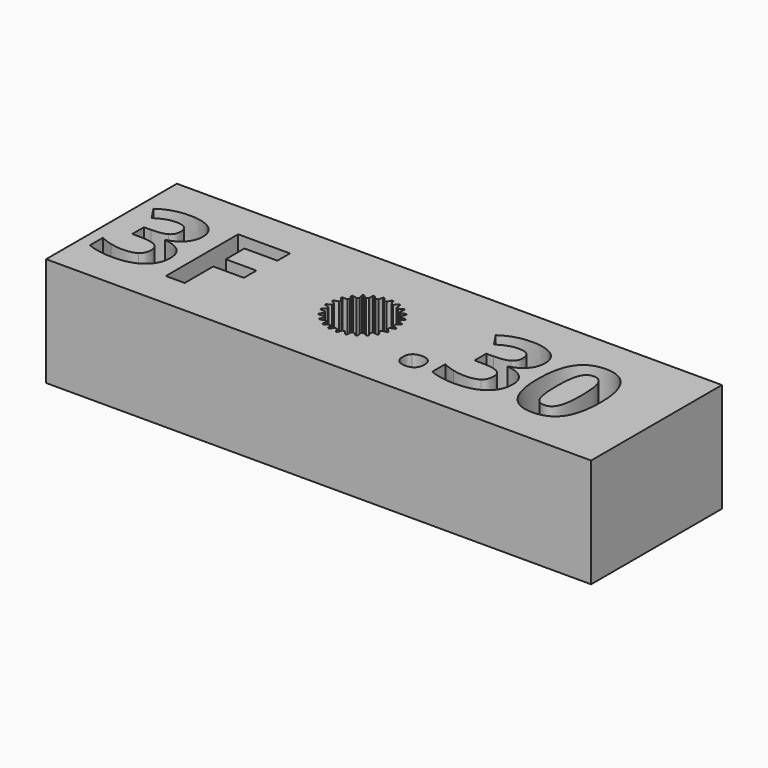
from build123d import *

# Parameters (mm, degrees)
F0_W         = 50
F0_H         = 15
F1_DEPTH     = 10
F0_TEXT_SIZE = 11.6133715069
F2_DEPTH     = 7


# Not quite as in the source:
# - a feature names something its author has since deleted; it is built from what else it names
# - Text() gives the source's letters only with a copy of the font that has no kerning and outlines rounded to 1/6400 em; it was checked with that copy


with BuildPart() as f1:
    # F0 (on Top) → F1 (new body)
    with BuildSketch(Plane.XY):
        with Locations((1.8412548097, 0.1652391267)):
            Rectangle(F0_W, F0_H)
        with BuildLine():
            add(Edge.make_bspline(
                [(-17.3084600185, 3.8715377677), (-16.5626638171, 3.3498433446), (-16.5626638171, 2.420773624)],
                knots=[0, 0, 0, 1, 1, 1], degree=2))
            add(Edge.make_bspline(
                [(-16.5626638171, 2.420773624), (-16.5626638171, 1.6441294045), (-17.0335497399, 1.0997526151)],
                knots=[0, 0, 0, 1, 1, 1], degree=2))
            add(Edge.make_bspline(
                [(-17.0335497399, 1.0997526151), (-17.5044356627, 0.5553758257), (-18.3554780435, 0.3503272351)],
                knots=[0, 0, 0, 1, 1, 1], degree=2))
            Line((-18.3554780435, 0.3503272351), (-18.3554780435, 0.3176646277))
            add(Edge.make_bspline(
                [(-18.3554780435, 0.3176646277), (-17.3501955724, 0.1924579661), (-16.8348522118, -0.2929446711)],
                knots=[0, 0, 0, 1, 1, 1], degree=2))
            add(Edge.make_bspline(
                [(-16.8348522118, -0.2929446711), (-16.3195088512, -0.7783473083), (-16.3195088512, -1.6003562602)],
                knots=[0, 0, 0, 1, 1, 1], degree=2))
            add(Edge.make_bspline(
                [(-16.3195088512, -1.6003562602), (-16.3195088512, -2.7961706076), (-17.1868825356, -3.4630321746)],
                knots=[0, 0, 0, 1, 1, 1], degree=2))
            add(Edge.make_bspline(
                [(-17.1868825356, -3.4630321746), (-18.05425622, -4.1298937416), (-19.6637969273, -4.1298937416)],
                knots=[0, 0, 0, 1, 1, 1], degree=2))
            add(Edge.make_bspline(
                [(-19.6637969273, -4.1298937416), (-21.013851365, -4.1298937416), (-22.0572402113, -3.681690185)],
                knots=[0, 0, 0, 1, 1, 1], degree=2))
            Line((-22.0572402113, -3.681690185), (-22.0572402113, -2.1900977821))
            add(Edge.make_bspline(
                [(-22.0572402113, -2.1900977821), (-21.5763740473, -2.433252748), (-20.9975200613, -2.5865855437)],
                knots=[0, 0, 0, 1, 1, 1], degree=2))
            add(Edge.make_bspline(
                [(-20.9975200613, -2.5865855437), (-20.4186660752, -2.7399183394), (-19.8525142143, -2.7399183394)],
                knots=[0, 0, 0, 1, 1, 1], degree=2))
            add(Edge.make_bspline(
                [(-19.8525142143, -2.7399183394), (-18.9833259406, -2.7399183394), (-18.5695995806, -2.4450475784)],
                knots=[0, 0, 0, 1, 1, 1], degree=2))
            add(Edge.make_bspline(
                [(-18.5695995806, -2.4450475784), (-18.1558732207, -2.1501768175), (-18.1558732207, -1.4969246703)],
                knots=[0, 0, 0, 1, 1, 1], degree=2))
            add(Edge.make_bspline(
                [(-18.1558732207, -1.4969246703), (-18.1558732207, -0.9144415056), (-18.6322029114, -0.670379245)],
                knots=[0, 0, 0, 1, 1, 1], degree=2))
            add(Edge.make_bspline(
                [(-18.6322029114, -0.670379245), (-19.1085326021, -0.4263169845), (-20.1519214484, -0.4263169845)],
                knots=[0, 0, 0, 1, 1, 1], degree=2))
            Line((-20.1519214484, -0.4263169845), (-20.7815839348, -0.4263169845))
            Line((-20.7815839348, -0.4263169845), (-20.7815839348, 0.9182936853))
            Line((-20.7815839348, 0.9182936853), (-20.1410339127, 0.9182936853))
            add(Edge.make_bspline(
                [(-20.1410339127, 0.9182936853), (-19.1774869954, 0.9182936853), (-18.7320053228, 1.1705215977)],
                knots=[0, 0, 0, 1, 1, 1], degree=2))
            add(Edge.make_bspline(
                [(-18.7320053228, 1.1705215977), (-18.2865236501, 1.4227495102), (-18.2865236501, 2.0342661036)],
                knots=[0, 0, 0, 1, 1, 1], degree=2))
            add(Edge.make_bspline(
                [(-18.2865236501, 2.0342661036), (-18.2865236501, 2.9760379492), (-19.4660066938, 2.9760379492)],
                knots=[0, 0, 0, 1, 1, 1], degree=2))
            add(Edge.make_bspline(
                [(-19.4660066938, 2.9760379492), (-19.8742892859, 2.9760379492), (-20.2970885923, 2.8399437519)],
                knots=[0, 0, 0, 1, 1, 1], degree=2))
            add(Edge.make_bspline(
                [(-20.2970885923, 2.8399437519), (-20.7198878987, 2.7038495545), (-21.2352312593, 2.3699651237)],
                knots=[0, 0, 0, 1, 1, 1], degree=2))
            Line((-21.2352312593, 2.3699651237), (-22.0463526755, 3.5766670068))
            add(Edge.make_bspline(
                [(-22.0463526755, 3.5766670068), (-20.9122343643, 4.3932321909), (-19.3408000323, 4.3932321909)],
                knots=[0, 0, 0, 1, 1, 1], degree=2))
            add(Edge.make_bspline(
                [(-19.3408000323, 4.3932321909), (-18.05425622, 4.3932321909), (-17.3084600185, 3.8715377677)],
                knots=[0, 0, 0, 1, 1, 1], degree=2))
        make_face(mode=Mode.SUBTRACT)
        Polygon((-13.0986128473, -0.7384263437), (-13.0986128473, -4.0155746158), (-14.8279164482, -4.0155746158), (-14.8279164482, 4.2752838865), (-10.0755070769, 4.2752838865), (-10.0755070769, 2.834499984), (-13.0986128473, 2.834499984), (-13.0986128473, 0.696913791), (-10.2859994355, 0.696913791), (-10.2859994355, -0.7384263437), align=None, mode=Mode.SUBTRACT)
        with BuildLine():
            ThreePointArc((-0.2085844925, 2.742078137), (-0.1043674356, 2.7480188206), (0, 2.75))
            Line((0, 2.75), (0.2117798247, 3.1428727791))
            ThreePointArc((0.2117798247, 3.1428727791), (0.2764112295, 3.1378490773), (0.3409255665, 3.1314964088))
            Line((0.3409255665, 3.1314964088), (0.4798956754, 2.7078035639))
            ThreePointArc((0.4798956754, 2.7078035639), (0.5823159498, 2.6876398819), (0.6838971897, 2.6636036931))
            Line((0.6838971897, 2.6636036931), (0.9867270488, 2.9914661507))
            ThreePointArc((0.9867270488, 2.9914661507), (1.0480785954, 2.970527101), (1.1089862515, 2.94832995))
            Line((1.1089862515, 2.94832995), (1.1382222331, 2.5033877343))
            ThreePointArc((1.1382222331, 2.5033877343), (1.2324102824, 2.4583866449), (1.3248226038, 2.4098433701))
            Line((1.3248226038, 2.4098433701), (1.6996745836, 2.6520947023))
            ThreePointArc((1.6996745836, 2.6520947023), (1.7538913287, 2.6165559821), (1.8073652517, 2.5799090773))
            Line((1.8073652517, 2.5799090773), (1.7250301017, 2.1416748465))
            ThreePointArc((1.7250301017, 2.1416748465), (1.8050677444, 2.0746639337), (1.8825045413, 2.0046637254))
            Line((1.8825045413, 2.0046637254), (2.3058253134, 2.1460823899))
            ThreePointArc((2.3058253134, 2.1460823899), (2.3495006193, 2.0981770278), (2.3921808461, 2.049383029))
            Line((2.3921808461, 2.049383029), (2.2034479849, 1.6453926516))
            ThreePointArc((2.2034479849, 1.6453926516), (2.2643061615, 1.5605824575), (2.3219017951, 1.4735236862))
            Line((2.3219017951, 1.4735236862), (2.7670925584, 1.5052238283))
            ThreePointArc((2.7670925584, 1.5052238283), (2.7974821452, 1.4479618942), (2.8266869202, 1.3900867079))
            Line((2.8266869202, 1.3900867079), (2.5434151275, 1.045724385))
            ThreePointArc((2.5434151275, 1.045724385), (2.581269895, 0.9484438461), (2.6154054198, 0.8497967345))
            Line((2.6154054198, 0.8497967345), (3.0544932014, 0.7697865177))
            ThreePointArc((3.0544932014, 0.7697865177), (3.0696875795, 0.7067659897), (3.0835818592, 0.6434461265))
            Line((3.0835818592, 0.6434461265), (2.7235701435, 0.3803494094))
            ThreePointArc((2.7235701435, 0.3803494094), (2.7360429477, 0.2767110197), (2.7445735032, 0.1726739287))
            Line((2.7445735032, 0.1726739287), (3.1499688028, -0.0140193109))
            ThreePointArc((3.1499688028, -0.0140193109), (3.1490132537, -0.0788386213), (3.1467240094, -0.1436245414))
            Line((3.1467240094, -0.1436245414), (2.7325932309, -0.3089243183))
            ThreePointArc((2.7325932309, -0.3089243183), (2.7189003595, -0.4124085778), (2.7012899395, -0.5152986151))
            Line((2.7012899395, -0.5152986151), (3.0475202797, -0.7969442547))
            ThreePointArc((3.0475202797, -0.7969442547), (3.0304748438, -0.8594895118), (3.0121459172, -0.9216707511))
            Line((3.0121459172, -0.9216707511), (2.5699174358, -0.9787871951))
            ThreePointArc((2.5699174358, -0.9787871951), (2.5309192623, -1.0756150276), (2.4882743943, -1.1708930518))
            Line((2.4882743943, -1.1708930518), (2.7535848493, -1.5297942599))
            ThreePointArc((2.7535848493, -1.5297942599), (2.7215205542, -1.5861355153), (2.6883036192, -1.6418049979))
            Line((2.6883036192, -1.6418049979), (2.2457642767, -1.5871492726))
            ThreePointArc((2.2457642767, -1.5871492726), (2.1839111998, -1.6712366293), (2.1189114176, -1.7529159718))
            Line((2.1189114176, -1.7529159718), (2.2866315559, -2.1665216656))
            ThreePointArc((2.2866315559, -2.1665216656), (2.2415631192, -2.2131187909), (2.1955453178, -2.2587785986))
            Line((2.1955453178, -2.2587785986), (1.7805014888, -2.0957849242))
            ThreePointArc((1.7805014888, -2.0957849242), (1.6996799648, -2.1618482873), (1.6164094438, -2.2247967345))
            Line((1.6164094438, -2.2247967345), (1.6760007922, -2.6671185472))
            ThreePointArc((1.6760007922, -2.6671185472), (1.6207600295, -2.7010436736), (1.5648328296, -2.7338248326))
            Line((1.5648328296, -2.7338248326), (1.203363244, -2.4727347013))
            ThreePointArc((1.203363244, -2.4727347013), (1.1086515866, -2.5166230666), (1.0123425199, -2.5568853362))
            Line((1.0123425199, -2.5568853362), (0.9600607348, -3.0001305614))
            ThreePointArc((0.9600607348, -3.0001305614), (0.8981186263, -3.0192520486), (0.8357961395, -3.0370947982))
            Line((0.8357961395, -3.0370947982), (0.5506132611, -2.694313463))
            ThreePointArc((0.5506132611, -2.694313463), (0.4479625518, -2.7132691632), (0.3446663923, -2.7283154286))
            Line((0.3446663923, -2.7283154286), (0.1837965306, -3.1446333388))
            ThreePointArc((0.1837965306, -3.1446333388), (0.1190451269, -3.1477497133), (0.0542433042, -3.1495329279))
            Line((0.0542433042, -3.1495329279), (-0.1367337781, -2.7465986008))
            ThreePointArc((-0.1367337781, -2.7465986008), (-0.2408736175, -2.7394305796), (-0.3446663923, -2.7283154286))
            Line((-0.3446663923, -2.7283154286), (-0.6040162856, -3.0915472383))
            ThreePointArc((-0.6040162856, -3.0915472383), (-0.6675084157, -3.078462687), (-0.7307178374, -3.0640743206))
            Line((-0.7307178374, -3.0640743206), (-0.8154893312, -2.6263048473))
            ThreePointArc((-0.8154893312, -2.6263048473), (-0.9145748116, -2.5934634977), (-1.0123425199, -2.5568853362))
            Line((-1.0123425199, -2.5568853362), (-1.3538765371, -2.844207855))
            ThreePointArc((-1.3538765371, -2.844207855), (-1.4121199496, -2.8157445282), (-1.4697652899, -2.7860886548))
            Line((-1.4697652899, -2.7860886548), (-1.4430046904, -2.3409907013))
            ThreePointArc((-1.4430046904, -2.3409907013), (-1.5308099067, -2.2845395662), (-1.6164094438, -2.2247967345))
            Line((-1.6164094438, -2.2247967345), (-2.0186677466, -2.4181564318))
            ThreePointArc((-2.0186677466, -2.4181564318), (-2.0680027937, -2.3761027851), (-2.1164619838, -2.3330427924))
            Line((-2.1164619838, -2.3330427924), (-1.9798507579, -1.9085835))
            ThreePointArc((-1.9798507579, -1.9085835), (-2.0508585855, -1.8320696117), (-2.1189114176, -1.7529159718))
            Line((-2.1189114176, -1.7529159718), (-2.5566186375, -1.8401633467))
            ThreePointArc((-2.5566186375, -1.8401633467), (-2.5939454167, -1.7871617653), (-2.6301735875, -1.733403271))
            Line((-2.6301735875, -1.733403271), (-2.3922955209, -1.3562529781))
            ThreePointArc((-2.3922955209, -1.3562529781), (-2.4420442768, -1.2644839857), (-2.4882743943, -1.1708930518))
            Line((-2.4882743943, -1.1708930518), (-2.9339277767, -1.1465460309))
            ThreePointArc((-2.9339277767, -1.1465460309), (-2.9569009092, -1.0859267991), (-2.9786217115, -1.024847647))
            Line((-2.9786217115, -1.024847647), (-2.6544235581, -0.7187040937))
            ThreePointArc((-2.6544235581, -0.7187040937), (-2.679787345, -0.6174461804), (-2.7012899395, -0.5152986151))
            Line((-2.7012899395, -0.5152986151), (-3.1268874436, -0.3808870112))
            ThreePointArc((-3.1268874436, -0.3808870112), (-3.1340634429, -0.3164590584), (-3.1399120789, -0.2518970763))
            Line((-3.1399120789, -0.2518970763), (-2.7497644008, -0.0359963878))
            ThreePointArc((-2.7497644008, -0.0359963878), (-2.7491495187, 0.0683880392), (-2.7445735032, 0.1726739287))
            Line((-2.7445735032, 0.1726739287), (-3.1233732724, 0.4087045402))
            ThreePointArc((-3.1233732724, 0.4087045402), (-3.1143012443, 0.4728929689), (-3.1039102225, 0.5368811142))
            Line((-3.1039102225, 0.5368811142), (-2.6723274333, 0.6489731035))
            ThreePointArc((-2.6723274333, 0.6489731035), (-2.6457725175, 0.7499251868), (-2.6154054198, 0.8497967345))
            Line((-2.6154054198, 0.8497967345), (-2.9236060716, 1.1726156822))
            ThreePointArc((-2.9236060716, 1.1726156822), (-2.8988560448, 1.2325313917), (-2.8728782714, 1.2919250897))
            Line((-2.8728782714, 1.2919250897), (-2.4269783051, 1.2931652279))
            ThreePointArc((-2.4269783051, 1.2931652279), (-2.3761518985, 1.3843417768), (-2.3219017951, 1.4735236862))
            Line((-2.3219017951, 1.4735236862), (-2.540137949, 1.8628470683))
            ThreePointArc((-2.540137949, 1.8628470683), (-2.5012650588, 1.9147253343), (-2.4613328129, 1.9657926605))
            Line((-2.4613328129, 1.9657926605), (-2.0291332041, 1.8561030252))
            ThreePointArc((-2.0291332041, 1.8561030252), (-1.9572289169, 1.9317750818), (-1.8825045413, 2.0046637254))
            Line((-1.8825045413, 2.0046637254), (-1.9970636172, 2.436028922))
            ThreePointArc((-1.9970636172, 2.436028922), (-1.9465103901, 2.4766100422), (-1.8951327616, 2.5161422488))
            Line((-1.8951327616, 2.5161422488), (-1.5037902013, 2.3024150431))
            ThreePointArc((-1.5037902013, 2.3024150431), (-1.4153260443, 2.3578278538), (-1.3248226038, 2.4098433701))
            Line((-1.3248226038, 2.4098433701), (-1.3285064335, 2.8561461195))
            ThreePointArc((-1.3285064335, 2.8561461195), (-1.2694493149, 2.8828802328), (-1.209854549, 2.9083933658))
            Line((-1.209854549, 2.9083933658), (-0.8839585296, 2.6040578561))
            ThreePointArc((-0.8839585296, 2.6040578561), (-0.7844930311, 2.6357296303), (-0.6838971897, 2.6636036931))
            Line((-0.6838971897, 2.6636036931), (-0.5764743048, 3.0968011521))
            ThreePointArc((-0.5764743048, 3.0968011521), (-0.5126240705, 3.108008456), (-0.4485567256, 3.1178994313))
            Line((-0.4485567256, 3.1178994313), (-0.2085844925, 2.742078137))
        make_face(mode=Mode.SUBTRACT)
        with BuildLine():
            add(Edge.make_bspline(
                [(6.516190169, -3.9157722044), (6.2557966047, -3.663544292), (6.2557966047, -3.2044531996)],
                knots=[0, 0, 0, 1, 1, 1], degree=2))
            add(Edge.make_bspline(
                [(6.2557966047, -3.2044531996), (6.2557966047, -2.7290308036), (6.5107464011, -2.484968543)],
                knots=[0, 0, 0, 1, 1, 1], degree=2))
            add(Edge.make_bspline(
                [(6.5107464011, -2.484968543), (6.7656961974, -2.2409062824), (7.2538207186, -2.2409062824)],
                knots=[0, 0, 0, 1, 1, 1], degree=2))
            add(Edge.make_bspline(
                [(7.2538207186, -2.2409062824), (7.7237993467, -2.2409062824), (7.9814710271, -2.4904123109)],
                knots=[0, 0, 0, 1, 1, 1], degree=2))
            add(Edge.make_bspline(
                [(7.9814710271, -2.4904123109), (8.2391427074, -2.7399183394), (8.2391427074, -3.2044531996)],
                knots=[0, 0, 0, 1, 1, 1], degree=2))
            add(Edge.make_bspline(
                [(8.2391427074, -3.2044531996), (8.2391427074, -3.6526567562), (7.9787491431, -3.9103284365)],
                knots=[0, 0, 0, 1, 1, 1], degree=2))
            add(Edge.make_bspline(
                [(7.9787491431, -3.9103284365), (7.7183555789, -4.1680001168), (7.2538207186, -4.1680001168)],
                knots=[0, 0, 0, 1, 1, 1], degree=2))
            add(Edge.make_bspline(
                [(7.2538207186, -4.1680001168), (6.7765837332, -4.1680001168), (6.516190169, -3.9157722044)],
                knots=[0, 0, 0, 1, 1, 1], degree=2))
        make_face(mode=Mode.SUBTRACT)
        with BuildLine():
            add(Edge.make_bspline(
                [(14.0948223719, 3.8715377677), (14.8406185733, 3.3498433446), (14.8406185733, 2.420773624)],
                knots=[0, 0, 0, 1, 1, 1], degree=2))
            add(Edge.make_bspline(
                [(14.8406185733, 2.420773624), (14.8406185733, 1.6441294045), (14.3697326505, 1.0997526151)],
                knots=[0, 0, 0, 1, 1, 1], degree=2))
            add(Edge.make_bspline(
                [(14.3697326505, 1.0997526151), (13.8988467277, 0.5553758257), (13.0478043469, 0.3503272351)],
                knots=[0, 0, 0, 1, 1, 1], degree=2))
            Line((13.0478043469, 0.3503272351), (13.0478043469, 0.3176646277))
            add(Edge.make_bspline(
                [(13.0478043469, 0.3176646277), (14.053086818, 0.1924579661), (14.5684301786, -0.2929446711)],
                knots=[0, 0, 0, 1, 1, 1], degree=2))
            add(Edge.make_bspline(
                [(14.5684301786, -0.2929446711), (15.0837735393, -0.7783473083), (15.0837735393, -1.6003562602)],
                knots=[0, 0, 0, 1, 1, 1], degree=2))
            add(Edge.make_bspline(
                [(15.0837735393, -1.6003562602), (15.0837735393, -2.7961706076), (14.2163998548, -3.4630321746)],
                knots=[0, 0, 0, 1, 1, 1], degree=2))
            add(Edge.make_bspline(
                [(14.2163998548, -3.4630321746), (13.3490261704, -4.1298937416), (11.7394854631, -4.1298937416)],
                knots=[0, 0, 0, 1, 1, 1], degree=2))
            add(Edge.make_bspline(
                [(11.7394854631, -4.1298937416), (10.3894310254, -4.1298937416), (9.3460421791, -3.681690185)],
                knots=[0, 0, 0, 1, 1, 1], degree=2))
            Line((9.3460421791, -3.681690185), (9.3460421791, -2.1900977821))
            add(Edge.make_bspline(
                [(9.3460421791, -2.1900977821), (9.8269083431, -2.433252748), (10.4057623291, -2.5865855437)],
                knots=[0, 0, 0, 1, 1, 1], degree=2))
            add(Edge.make_bspline(
                [(10.4057623291, -2.5865855437), (10.9846163152, -2.7399183394), (11.5507681761, -2.7399183394)],
                knots=[0, 0, 0, 1, 1, 1], degree=2))
            add(Edge.make_bspline(
                [(11.5507681761, -2.7399183394), (12.4199564499, -2.7399183394), (12.8336828098, -2.4450475784)],
                knots=[0, 0, 0, 1, 1, 1], degree=2))
            add(Edge.make_bspline(
                [(12.8336828098, -2.4450475784), (13.2474091697, -2.1501768175), (13.2474091697, -1.4969246703)],
                knots=[0, 0, 0, 1, 1, 1], degree=2))
            add(Edge.make_bspline(
                [(13.2474091697, -1.4969246703), (13.2474091697, -0.9144415056), (12.771079479, -0.670379245)],
                knots=[0, 0, 0, 1, 1, 1], degree=2))
            add(Edge.make_bspline(
                [(12.771079479, -0.670379245), (12.2947497883, -0.4263169845), (11.251360942, -0.4263169845)],
                knots=[0, 0, 0, 1, 1, 1], degree=2))
            Line((11.251360942, -0.4263169845), (10.6216984556, -0.4263169845))
            Line((10.6216984556, -0.4263169845), (10.6216984556, 0.9182936853))
            Line((10.6216984556, 0.9182936853), (11.2622484778, 0.9182936853))
            add(Edge.make_bspline(
                [(11.2622484778, 0.9182936853), (12.225795395, 0.9182936853), (12.6712770676, 1.1705215977)],
                knots=[0, 0, 0, 1, 1, 1], degree=2))
            add(Edge.make_bspline(
                [(12.6712770676, 1.1705215977), (13.1167587403, 1.4227495102), (13.1167587403, 2.0342661036)],
                knots=[0, 0, 0, 1, 1, 1], degree=2))
            add(Edge.make_bspline(
                [(13.1167587403, 2.0342661036), (13.1167587403, 2.9760379492), (11.9372756966, 2.9760379492)],
                knots=[0, 0, 0, 1, 1, 1], degree=2))
            add(Edge.make_bspline(
                [(11.9372756966, 2.9760379492), (11.5289931046, 2.9760379492), (11.1061937981, 2.8399437519)],
                knots=[0, 0, 0, 1, 1, 1], degree=2))
            add(Edge.make_bspline(
                [(11.1061937981, 2.8399437519), (10.6833944917, 2.7038495545), (10.1680511311, 2.3699651237)],
                knots=[0, 0, 0, 1, 1, 1], degree=2))
            Line((10.1680511311, 2.3699651237), (9.3569297149, 3.5766670068))
            add(Edge.make_bspline(
                [(9.3569297149, 3.5766670068), (10.4910480261, 4.3932321909), (12.0624823582, 4.3932321909)],
                knots=[0, 0, 0, 1, 1, 1], degree=2))
            add(Edge.make_bspline(
                [(12.0624823582, 4.3932321909), (13.3490261704, 4.3932321909), (14.0948223719, 3.8715377677)],
                knots=[0, 0, 0, 1, 1, 1], degree=2))
        make_face(mode=Mode.SUBTRACT)
        with BuildLine():
            add(Edge.make_bspline(
                [(21.0129440703, 3.3171807372), (21.7469454413, 2.2284271584), (21.7469454413, 0.1289473407)],
                knots=[0, 0, 0, 1, 1, 1], degree=2))
            add(Edge.make_bspline(
                [(21.7469454413, 0.1289473407), (21.7469454413, -2.0413014596), (21.0356264365, -3.0855976006)],
                knots=[0, 0, 0, 1, 1, 1], degree=2))
            add(Edge.make_bspline(
                [(21.0356264365, -3.0855976006), (20.3243074318, -4.1298937416), (18.8436025646, -4.1298937416)],
                knots=[0, 0, 0, 1, 1, 1], degree=2))
            add(Edge.make_bspline(
                [(18.8436025646, -4.1298937416), (17.4082624299, -4.1298937416), (16.6797048268, -3.0520276986)],
                knots=[0, 0, 0, 1, 1, 1], degree=2))
            add(Edge.make_bspline(
                [(16.6797048268, -3.0520276986), (15.9511472237, -1.9741616556), (15.9511472237, 0.1289473407)],
                knots=[0, 0, 0, 1, 1, 1], degree=2))
            add(Edge.make_bspline(
                [(15.9511472237, 0.1289473407), (15.9511472237, 2.3246003912), (16.6606516392, 3.3652673536)],
                knots=[0, 0, 0, 1, 1, 1], degree=2))
            add(Edge.make_bspline(
                [(16.6606516392, 3.3652673536), (17.3701560547, 4.405934316), (18.8436025646, 4.405934316)],
                knots=[0, 0, 0, 1, 1, 1], degree=2))
            add(Edge.make_bspline(
                [(18.8436025646, 4.405934316), (20.2789426993, 4.405934316), (21.0129440703, 3.3171807372)],
                knots=[0, 0, 0, 1, 1, 1], degree=2))
        make_face(mode=Mode.SUBTRACT)
    extrude(amount=F1_DEPTH)



with BuildPart() as f1b:
    # F0 (on Top) → F1, piece 2 (new body)
    with BuildSketch(Plane.XY):
        with BuildLine():
            add(Edge.make_bspline(
                [(17.9589902819, 2.3209712126), (17.6931529497, 1.6550169403), (17.6931529497, 0.1289473407)],
                knots=[0, 0, 0, 1, 1, 1], degree=2))
            add(Edge.make_bspline(
                [(17.6931529497, 0.1289473407), (17.6931529497, -1.3953076696), (17.9562683979, -2.055818174)],
                knots=[0, 0, 0, 1, 1, 1], degree=2))
            add(Edge.make_bspline(
                [(17.9562683979, -2.055818174), (18.2193838461, -2.7163286785), (18.8436025646, -2.7163286785)],
                knots=[0, 0, 0, 1, 1, 1], degree=2))
            add(Edge.make_bspline(
                [(18.8436025646, -2.7163286785), (19.4569337473, -2.7163286785), (19.729122142, -2.0476525222)],
                knots=[0, 0, 0, 1, 1, 1], degree=2))
            add(Edge.make_bspline(
                [(19.729122142, -2.0476525222), (20.0013105367, -1.3789763659), (20.0013105367, 0.1289473407)],
                knots=[0, 0, 0, 1, 1, 1], degree=2))
            add(Edge.make_bspline(
                [(20.0013105367, 0.1289473407), (20.0013105367, 1.6550169403), (19.7254929634, 2.3209712126)],
                knots=[0, 0, 0, 1, 1, 1], degree=2))
            add(Edge.make_bspline(
                [(19.7254929634, 2.3209712126), (19.4496753901, 2.986925485), (18.8436025646, 2.986925485)],
                knots=[0, 0, 0, 1, 1, 1], degree=2))
            add(Edge.make_bspline(
                [(18.8436025646, 2.986925485), (18.224827614, 2.986925485), (17.9589902819, 2.3209712126)],
                knots=[0, 0, 0, 1, 1, 1], degree=2))
        make_face()
    extrude(amount=F1_DEPTH)


with BuildPart() as f1_1:
    add(f1.part)

    add(f1b.part)  # F2 merges F1b
    # F0 (on Top) → F2 (join)
    with BuildSketch(Plane.XY):
        with Locations((-22.5, -4.0155746158)):
            Text('3F     .30', F0_TEXT_SIZE, font='Open Sans', font_style=FontStyle.BOLD, text_align=(TextAlign.LEFT, TextAlign.BOTTOM))
    extrude(amount=F2_DEPTH)


solid = f1_1.part
